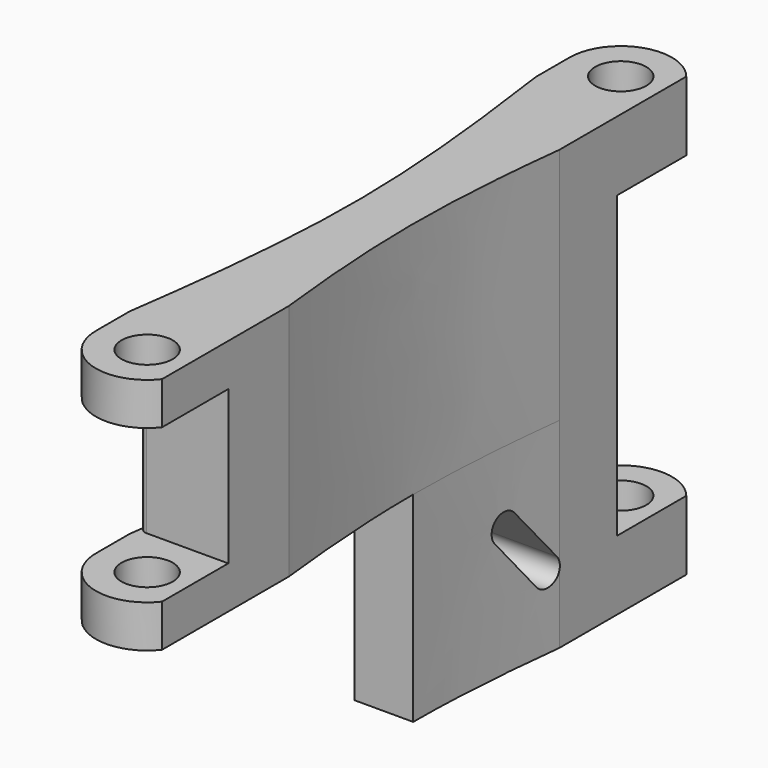
from build123d import *

# Parameters (mm, degrees)
F0_R     = 1.75
F1_DEPTH = 16.3
F2_W     = 0.6277186767
F2_H     = 10.5
F2_W_2   = 2.8722813233
F2_W_3   = 3.5
F3_DEPTH = 25
F4_DEPTH = 13.7
F5_W     = 3.75
F5_H     = 20.5
F6_DEPTH = 25
F7_R     = 0.5
F9_DEPTH = 44


# Not quite as in the source:
# - a feature names something its author has since deleted; it is built from what else it names


with BuildPart() as f1:
    # F0 (on Top) → F1 (new body)
    with BuildSketch(Plane.XY):
        with BuildLine():
            ThreePointArc((-3.5, 0), (0, -3.5), (3.5, 0))
            ThreePointArc((3.5, 0), (0, 3.5), (-3.5, 0))
        make_face()
        Circle(F0_R, mode=Mode.SUBTRACT)
        with BuildLine():
            ThreePointArc((-3.5, 40.5), (0, 37), (3.5, 40.5))
            ThreePointArc((3.5, 40.5), (0, 44), (-3.5, 40.5))
        make_face()
        with Locations((0, 40.5)):
            Circle(F0_R, mode=Mode.SUBTRACT)
        with BuildLine():
            Line((-2, 20.25), (2, 20.25))
            add(Edge.make_bspline(
                [(3.5, 37.6277186767), (2.75, 32.25), (2, 26.25), (2, 20.25)],
                knots=[0, 0, 0, 0, 0.5, 0.5, 0.5, 0.5], degree=3))
            Line((3.5, 37.6277186767), (3.5, 40.5))
            ThreePointArc((3.5, 40.5), (0, 37), (-3.5, 40.5))
            Line((-3.5, 40.5), (-3.5, 37.6277186767))
            add(Edge.make_bspline(
                [(-3.5, 37.6277186767), (-2.75, 32.25), (-2, 26.25), (-2, 20.25)],
                knots=[0, 0, 0, 0, 0.5, 0.5, 0.5, 0.5], degree=3))
        make_face()
        with BuildLine():
            ThreePointArc((-3.5, 0), (0, 3.5), (3.5, 0))
            Line((3.5, 0), (3.5, 2.8722813233))
            add(Edge.make_bspline(
                [(2, 20.25), (2, 14.25), (2.75, 8.25), (3.5, 2.8722813233)],
                knots=[0.5, 0.5, 0.5, 0.5, 1, 1, 1, 1], degree=3))
            Line((2, 20.25), (-2, 20.25))
            add(Edge.make_bspline(
                [(-2, 20.25), (-2, 14.25), (-2.75, 8.25), (-3.5, 2.8722813233)],
                knots=[0.5, 0.5, 0.5, 0.5, 1, 1, 1, 1], degree=3))
            Line((-3.5, 2.8722813233), (-3.5, 0))
        make_face()
    extrude(amount=F1_DEPTH)

    # F2 (on face) → F3 (cut)
    with BuildSketch(Plane(origin=(-3.5, 0, 0), x_dir=(0, -1, 0), z_dir=(-1, 0, 0))):
        with Locations((-3.1861406616, 8.15)):
            Rectangle(F2_W, F2_H)
        with Locations((-1.4361406616, 8.15)):
            Rectangle(F2_W_2, F2_H)
        with Locations((1.75, 8.15)):
            Rectangle(F2_W_3, F2_H)
    extrude(amount=-F3_DEPTH, mode=Mode.SUBTRACT)

    # F0 (on Top) → F4 (join)
    with BuildSketch(Plane.XY):
        with BuildLine():
            ThreePointArc((-3.5, 40.5), (0, 37), (3.5, 40.5))
            ThreePointArc((3.5, 40.5), (0, 44), (-3.5, 40.5))
        make_face()
        with Locations((0, 40.5)):
            Circle(F0_R, mode=Mode.SUBTRACT)
        with BuildLine():
            Line((-2, 20.25), (2, 20.25))
            add(Edge.make_bspline(
                [(3.5, 37.6277186767), (2.75, 32.25), (2, 26.25), (2, 20.25)],
                knots=[0, 0, 0, 0, 0.5, 0.5, 0.5, 0.5], degree=3))
            Line((3.5, 37.6277186767), (3.5, 40.5))
            ThreePointArc((3.5, 40.5), (0, 37), (-3.5, 40.5))
            Line((-3.5, 40.5), (-3.5, 37.6277186767))
            add(Edge.make_bspline(
                [(-3.5, 37.6277186767), (-2.75, 32.25), (-2, 26.25), (-2, 20.25)],
                knots=[0, 0, 0, 0, 0.5, 0.5, 0.5, 0.5], degree=3))
        make_face()
    extrude(amount=-F4_DEPTH)

    # F5 (on face) → F6 (cut)
    with BuildSketch(Plane(origin=(-3.5, 0, 0), x_dir=(0, -1, 0), z_dir=(-1, 0, 0))):
        with Locations((-42.375, 1.3)):
            Rectangle(F5_W, F5_H)
        Polygon((-37.6277186767, 0), (-37.6277186767, 11.55), (-40.5, 11.55), (-40.5, -8.95), (-37.6277186767, -8.95), align=None)
        Polygon((-36.75, -8.95), (-36.75, 11.55), (-37.6277186767, 11.55), (-37.6277186767, 0), (-37.6277186767, -8.95), align=None)
        with BuildLine():
            ThreePointArc((-30.0909245811, -9.4078987175), (-29.9172764034, -9.1071312511), (-29.8569690242, -8.7651111078))
            ThreePointArc((-29.8569690242, -8.7651111078), (-30.5149488809, -7.825418487), (-31.6230134673, -8.1223234981))
            ThreePointArc((-31.6230134673, -8.1223234981), (-31.4997566339, -9.5311555509), (-30.0909245811, -9.4078987175))
        make_face()
        with BuildLine():
            ThreePointArc((-31.6230134673, -8.1223234981), (-30.5149488809, -7.825418487), (-29.8569690242, -8.7651111078))
            ThreePointArc((-29.8569690242, -8.7651111078), (-29.9172764034, -9.1071312511), (-30.0909245811, -9.4078987175))
            Line((-30.0909245811, -9.4078987175), (-26.8769865327, -5.5776765019))
            ThreePointArc((-26.8769865327, -5.5776765019), (-28.2858185855, -5.7009333353), (-28.4090754189, -4.2921012825))
            Line((-28.4090754189, -4.2921012825), (-31.6230134673, -8.1223234981))
        make_face()
        with BuildLine():
            ThreePointArc((-26.6430309758, -4.9348888922), (-27.3010108325, -3.9951962714), (-28.4090754189, -4.2921012825))
            ThreePointArc((-28.4090754189, -4.2921012825), (-28.2858185855, -5.7009333353), (-26.8769865327, -5.5776765019))
            ThreePointArc((-26.8769865327, -5.5776765019), (-26.703338355, -5.2769090355), (-26.6430309758, -4.9348888922))
        make_face()
    extrude(amount=-F6_DEPTH, mode=Mode.SUBTRACT)

    # F7
    f7_edges = [f1.edges().sort_by_distance(p)[0] for p in [
        (-3.412885, 3.5, 8.15),
        (3.412885, 3.5, 8.15),
        (3.378456, 36.75, 5.775),
        (3.378456, 36.75, -4.475),
        (-3.378456, 36.75, 5.775),
        (-3.378456, 36.75, -4.475),
    ]]
    fillet(f7_edges, radius=F7_R)

    # F8 (on face) → F9 (cut)
    with BuildSketch(Plane.XY.offset(16.3)):
        with BuildLine():
            ThreePointArc((3.5, 40.5), (3.3071891388, 41.6456439237), (2.75, 42.6650635095))
            Line((2.75, 42.6650635095), (2.75, 31.8256302364))
            add(Edge.make_bspline(
                [(2.75, 31.8256302364), (2.979055467, 33.8173381724), (3.2395277335, 35.7600565803), (3.5, 37.6277186767)],
                knots=[1.3263518223, 1.3263518223, 1.3263518223, 1.3263518223, 1.5, 1.5, 1.5, 1.5], degree=3))
            Line((3.5, 37.6277186767), (3.5, 40.5))
        make_face()
        with BuildLine():
            add(Edge.make_bspline(
                [(3.5, 2.8722813233), (3.2395277335, 4.7399434197), (2.979055467, 6.6826618276), (2.75, 8.6743697636)],
                knots=[0.5, 0.5, 0.5, 0.5, 0.6736481777, 0.6736481777, 0.6736481777, 0.6736481777], degree=3))
            Line((2.75, 8.6743697636), (2.75, -2.1650635095))
            ThreePointArc((2.75, -2.1650635095), (3.3071891388, -1.1456439237), (3.5, 0))
            Line((3.5, 0), (3.5, 2.8722813233))
        make_face()
    extrude(amount=-F9_DEPTH, mode=Mode.SUBTRACT)


solid = f1.part
